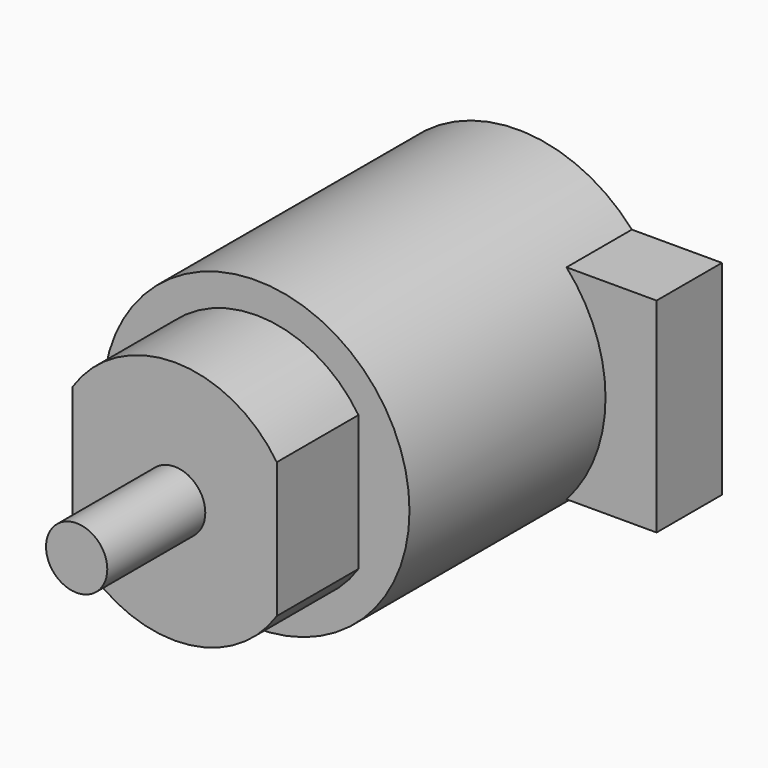
from build123d import *

# Parameters (mm, degrees)
F0_R     = 3.75
F1_DEPTH = 8
F3_DEPTH = 2.5
F4_R     = 0.75
F5_DEPTH = 3
F7_DEPTH = 2


# Not quite as in the source:
# - a feature names something its author has since deleted; it is built from what else it names


with BuildPart() as f1:
    # F0 (on Front) → F1 (new body)
    with BuildSketch(Plane.XZ):
        Circle(F0_R)
    extrude(amount=F1_DEPTH)

    # F2 (on face) → F3 (join)
    with BuildSketch(Plane.XZ.offset(8)):
        with BuildLine():
            Line((-2.5, 1.6583123952), (-2.5, -1.6583123952))
            ThreePointArc((-2.5, -1.6583123952), (0, -3), (2.5, -1.6583123952))
            Line((2.5, -1.6583123952), (2.5, 1.6583123952))
            ThreePointArc((2.5, 1.6583123952), (0, 3), (-2.5, 1.6583123952))
        make_face()
    extrude(amount=F3_DEPTH)

    # F4 (on face) → F5 (join)
    with BuildSketch(Plane.XZ.offset(10.5)):
        Circle(F4_R)
    extrude(amount=F5_DEPTH)

    # F6 (on face) → F7 (join)
    with BuildSketch(Plane(origin=(0, 0, 0), x_dir=(-1, 0, 0), z_dir=(0, 1, 0))):
        with BuildLine():
            Line((0, 2.5), (-2.7950849719, 2.5))
            ThreePointArc((-2.7950849719, 2.5), (-3.75, 0), (-2.7950849719, -2.5))
            Line((-2.7950849719, -2.5), (0, -2.5))
            Line((0, -2.5), (0, 2.5))
        make_face()
        with BuildLine():
            Line((-2.7950849719, 2.5), (-5, 2.5))
            Line((-5, 2.5), (-5, -2.5))
            Line((-5, -2.5), (-2.7950849719, -2.5))
            ThreePointArc((-2.7950849719, -2.5), (-3.75, 0), (-2.7950849719, 2.5))
        make_face()
    extrude(amount=-F7_DEPTH)


solid = f1.part
